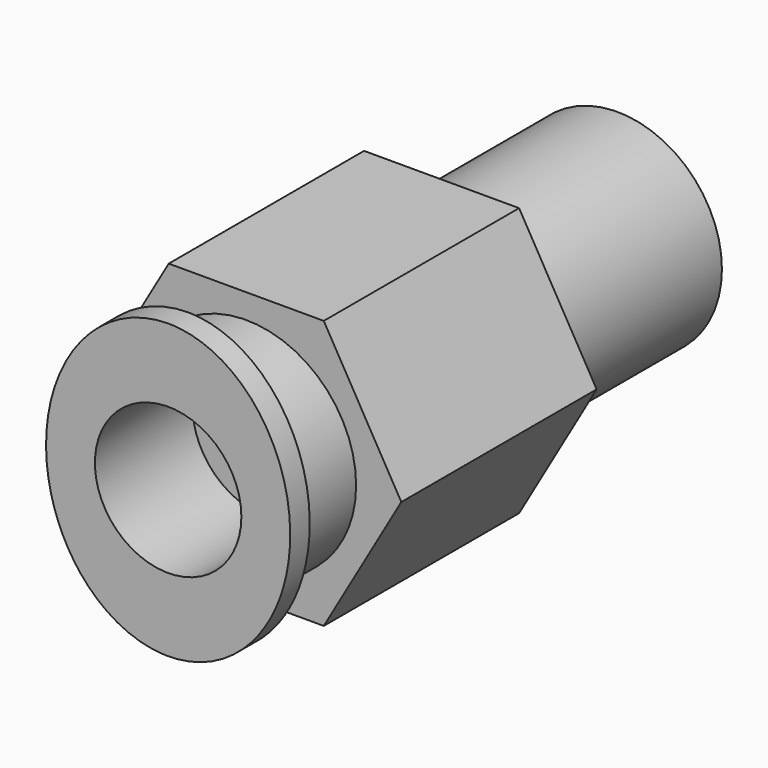
from build123d import *

# Parameters (mm, degrees)
F0_R     = 4.283
F1_DEPTH = 9
F2_R     = 4.283
F3_DEPTH = 10
F4_R     = 4.5
F5_DEPTH = 3
F7_DEPTH = 1
F8_R     = 3
F9_DEPTH = 5


# Not quite as in the source:
# - a feature names something its author has since deleted; it is built from what else it names


with BuildPart() as f1:
    # F0 (on Front) → F1 (new body)
    with BuildSketch(Plane.XZ):
        Circle(F0_R)
    extrude(amount=F1_DEPTH)

    # F2 (on face) → F3 (join)
    with BuildSketch(Plane.XZ.offset(9)):
        Polygon((3.1754264805, 5.5), (-3.1754264805, 5.5), (-6.3508529611, 0), (-3.1754264805, -5.5), (3.1754264805, -5.5), (6.3508529611, 0), align=None)
        Circle(F2_R, mode=Mode.SUBTRACT)
        Circle(F2_R)
    extrude(amount=F3_DEPTH)

    # F4 (on face) → F5 (join)
    with BuildSketch(Plane.XZ.offset(19)):
        Circle(F4_R)
    extrude(amount=F5_DEPTH)

    # F6 (on face) → F7 (join)
    with BuildSketch(Plane.XZ.offset(22)):
        with BuildLine():
            add(Edge.make_bspline(
                [(0, 6), (-8.6602540378, 6), (-4.3301270189, -3), (0, -12), (4.3301270189, -3), (8.6602540378, 6), (0, 6)],
                knots=[0, 0, 0, 2.0943951024, 2.0943951024, 4.1887902048, 4.1887902048, 6.2831853072, 6.2831853072, 6.2831853072], degree=2, weights=[1, 0.5, 1, 0.5, 1, 0.5, 1]))
        make_face()
    extrude(amount=F7_DEPTH)

    # F8 (on face) → F9 (cut)
    with BuildSketch(Plane.XZ.offset(23)):
        Circle(F8_R)
    extrude(amount=-F9_DEPTH, mode=Mode.SUBTRACT)


solid = f1.part
